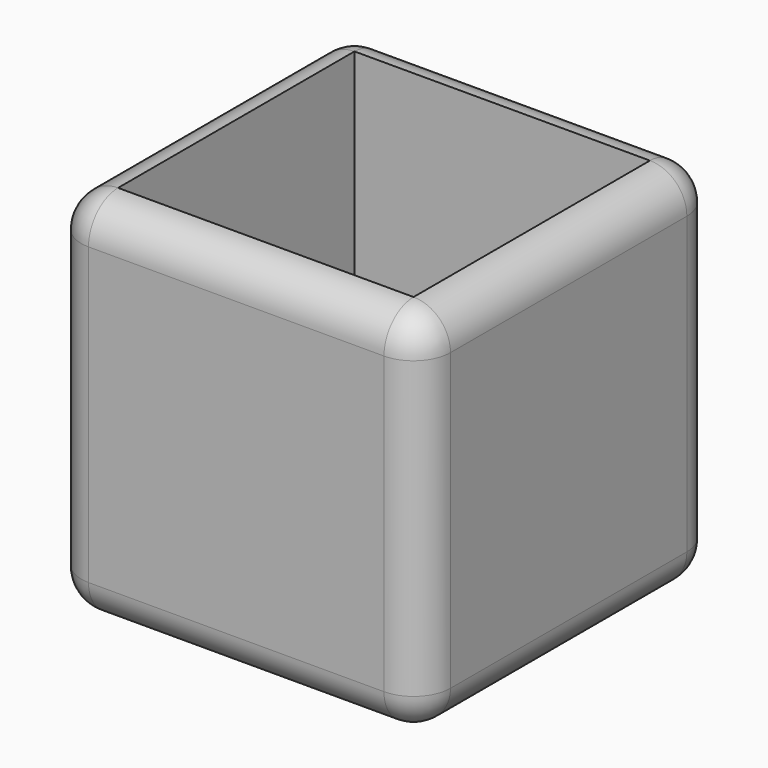
from build123d import *

# Parameters (mm, degrees)
F1_DEPTH = 20
F3_T     = 2
F4_R     = 1.99999


# Not quite as in the source:
# - a fillet or chamfer is up to 0.001 mm smaller than in the source, because OpenCascade refuses the exact size
# - a feature of the source that left no trace in its solid (it failed there, or was rolled back) is left out
# - a shell that OpenCascade refuses in one call is made with other operations: the cavity is built on its own and cut out


with BuildPart() as f1:
    # F0 (on Top) → F1 (new body)
    with BuildSketch(Plane.XY):
        with BuildLine():
            Line((-8, -10), (8, -10))
            ThreePointArc((8, -10), (9.4142135624, -9.4142135624), (10, -8))
            Line((10, -8), (10, 8))
            ThreePointArc((10, 8), (9.4142135624, 9.4142135624), (8, 10))
            Line((8, 10), (-8, 10))
            ThreePointArc((-8, 10), (-9.4142135624, 9.4142135624), (-10, 8))
            Line((-10, 8), (-10, -8))
            ThreePointArc((-10, -8), (-9.4142135624, -9.4142135624), (-8, -10))
        make_face()
    extrude(amount=F1_DEPTH)

    # F3: shell of thickness 2, made by hand


with BuildPart() as f3_core1:
    # F3_t2: copy of F1
    add(f1.part)

    # the walls: a layer under each face that stays
    f3_faces = [f3_core1.faces().sort_by_distance(p)[0] for p in [
        (0, -10, 10),
        (10, 0, 10),
        (0, 10, 10),
        (-10, 0, 10),
        (0, 0, 0),
    ]]
    thicken(f3_faces, amount=-F3_T, mode=Mode.SUBTRACT)


with BuildPart() as f1_1:
    add(f1.part)

    # what is left inside the walls is the cavity
    f3_cavity = [f3_core1.part.solids().sort_by_distance(p)[0] for p in [
        (0, -7.98, 14),
    ]]
    add(f3_cavity, mode=Mode.SUBTRACT)

    # F4 (radius 2 in the source; OpenCascade refuses exactly that, so slightly less here)
    f4_edges = [f1_1.edges().sort_by_distance(p)[0] for p in [
        (0, -10, 0),
        (0, -10, 20),
        (-9.414214, -9.414214, 0),
        (-9.414214, -9.414214, 20),
        (9.414214, -9.414214, 0),
        (9.414214, -9.414214, 20),
        (10, 0, 0),
        (9.414214, 9.414214, 0),
        (0, 10, 0),
        (-9.414214, 9.414214, 0),
        (-10, 0, 0),
        (-10, 0, 20),
        (10, 0, 20),
        (-9.414214, 9.414214, 20),
        (9.414214, 9.414214, 20),
        (0, 10, 20),
        (0, -8, 2),
        (8, 0, 2),
        (0, 8, 2),
        (-8, 0, 2),
    ]]
    fillet(f4_edges, radius=F4_R)


solid = f1_1.part
